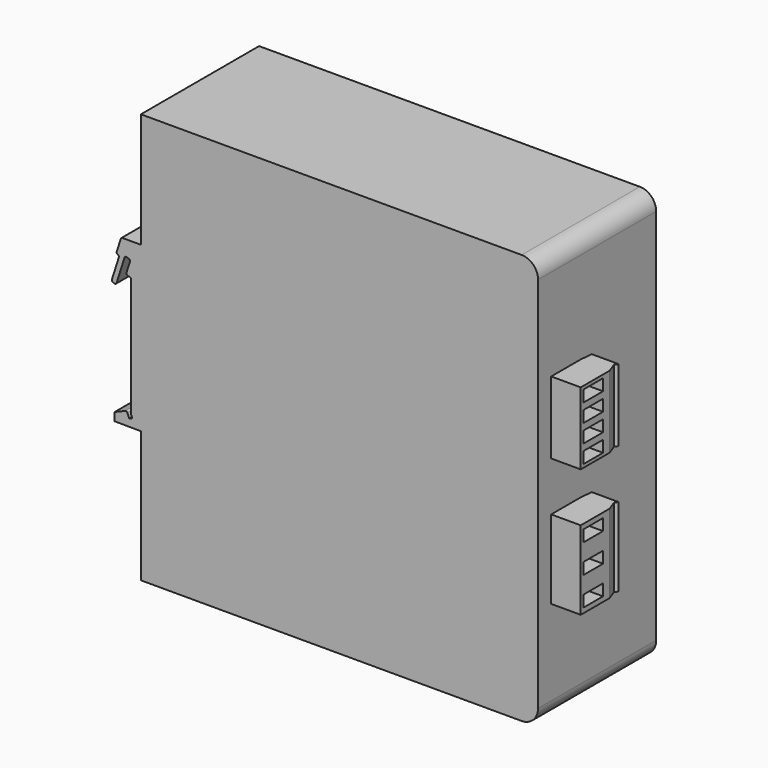
from build123d import *

# Parameters (mm, degrees)
F0_W      = 121
F0_H      = 45
F1_DEPTH  = 125
F2_R      = 5
F3_W      = 11
F3_H      = 22
F4_DEPTH  = 9
F3_H_2    = 24
F6_DEPTH  = 22
F8_DEPTH  = 24
F9_W      = 7.5
F9_H      = 3.5
F10_DEPTH = 5
F11_DEPTH = 5
F13_DEPTH = 45
F14_R     = 0.5
F15_R     = 0.49999


# Not quite as in the source:
# - a fillet or chamfer is up to 0.001 mm smaller than in the source, because OpenCascade refuses the exact size
# - a feature names something its author has since deleted; it is built from what else it names


with BuildPart() as f1:
    # F0 (on Top) → F1 (new body)
    with BuildSketch(Plane.XY):
        Rectangle(F0_W, F0_H)
    extrude(amount=F1_DEPTH)

    # F2
    f2_edges = [f1.edges().sort_by_distance(p)[0] for p in [
        (60.5, 0, 125),
        (60.5, 0, 0),
    ]]
    fillet(f2_edges, radius=F2_R)

    # F12 (on face) → F13 (join, through all)
    with BuildSketch(Plane(origin=(0, 22.5, 0), x_dir=(-1, 0, 0), z_dir=(0, 1, 0))):
        Polygon((60.5, 90), (60.5, 40), (68.4998644438, 40.0465712465), (68.4998644438, 42.5465712465), (64.8077652628, 44.0855331166), (64.0382843277, 42.2394835261), (63.1152595325, 42.6242239936), (63.5, 43.5472487889), (63.5, 80.1200936495), (65.0437947471, 80.6128124606), (63.6755676946, 84.8997641436), (65.3345620006, 85.4292501414), (68.0710161057, 76.8553467754), (69.5, 77.3114224596), (67.067596351, 84.9326698961), (68.0202522806, 85.2367203522), (66.5, 90), align=None)
    extrude(amount=-F13_DEPTH)

    # F14
    f14_edges = [f1.edges().sort_by_distance(p)[0] for p in [
        (-67.067596, 0, 84.93267),
        (-63.675568, 0, 84.899764),
        (-63.5, 0, 80.120094),
    ]]
    fillet(f14_edges, radius=F14_R)

    # F15 (radius 0.5 in the source; OpenCascade refuses exactly that, so slightly less here)
    f15_edges = [f1.edges().sort_by_distance(p)[0] for p in [
        (-68.020252, 0, 85.23672),
        (-69.5, 0, 77.311422),
        (-68.071016, 0, 76.855347),
        (-65.334562, 0, 85.42925),
        (-66.5, 0, 90),
        (-65.043795, 0, 80.612812),
        (-64.807765, 0, 44.085533),
        (-63.5, 0, 43.547249),
    ]]
    fillet(f15_edges, radius=F15_R)


with BuildPart() as f4:
    # F3 (on face) → F4 (new body)
    with BuildSketch(Plane.YZ.offset(60.5)):
        with Locations((-12, 81)):
            Rectangle(F3_W, F3_H)
    extrude(amount=F4_DEPTH)

    # F5 (on face) → F6 (join, through all)
    with BuildSketch(Plane(origin=(0, 0, 70), x_dir=(1, 0, 0), z_dir=(0, 0, -1))):
        Polygon((68.3861392063, 3.4396926208), (69.5, 6.5), (60.5, 6.5), (60.8499546541, 2.5), (68.0441190629, 2.5), align=None)
        Polygon((69.0441190629, 2.5), (68.3861392063, 3.4396926208), (68.0441190629, 2.5), align=None)
    extrude(amount=-F6_DEPTH)

    # F9 (on face) → F11 (cut)
    with BuildSketch(Plane.YZ.offset(69.5)):
        with Locations((-12.75, 72.75)):
            Rectangle(F9_W, F9_H)
        with Locations((-12.75, 78.25)):
            Rectangle(F9_W, F9_H)
        with Locations((-12.75, 83.75)):
            Rectangle(F9_W, F9_H)
        with Locations((-12.75, 89.25)):
            Rectangle(F9_W, F9_H)
    extrude(amount=-F11_DEPTH, mode=Mode.SUBTRACT)


with BuildPart() as f4b:
    # F3 (on face) → F4, piece 2 (new body)
    with BuildSketch(Plane.YZ.offset(60.5)):
        with Locations((-12, 43)):
            Rectangle(F3_W, F3_H_2)
    extrude(amount=F4_DEPTH)

    # F7 (on face) → F8 (join, through all)
    with BuildSketch(Plane(origin=(0, 0, 31), x_dir=(1, 0, 0), z_dir=(0, 0, -1))):
        Polygon((68.3861392063, 3.4396926208), (69.5, 6.5), (60.5, 6.5), (60.8499546541, 2.5), (68.0441190629, 2.5), align=None)
        Polygon((69.0441190629, 2.5), (68.3861392063, 3.4396926208), (68.0441190629, 2.5), align=None)
    extrude(amount=-F8_DEPTH)

    # F9 (on face) → F10 (cut)
    with BuildSketch(Plane.YZ.offset(69.5)):
        with Locations((-12.75, 34.25)):
            Rectangle(F9_W, F9_H)
        with Locations((-12.75, 43)):
            Rectangle(F9_W, F9_H)
        with Locations((-12.75, 51.75)):
            Rectangle(F9_W, F9_H)
    extrude(amount=-F10_DEPTH, mode=Mode.SUBTRACT)


solid = Compound([f1.part, f4.part, f4b.part])
